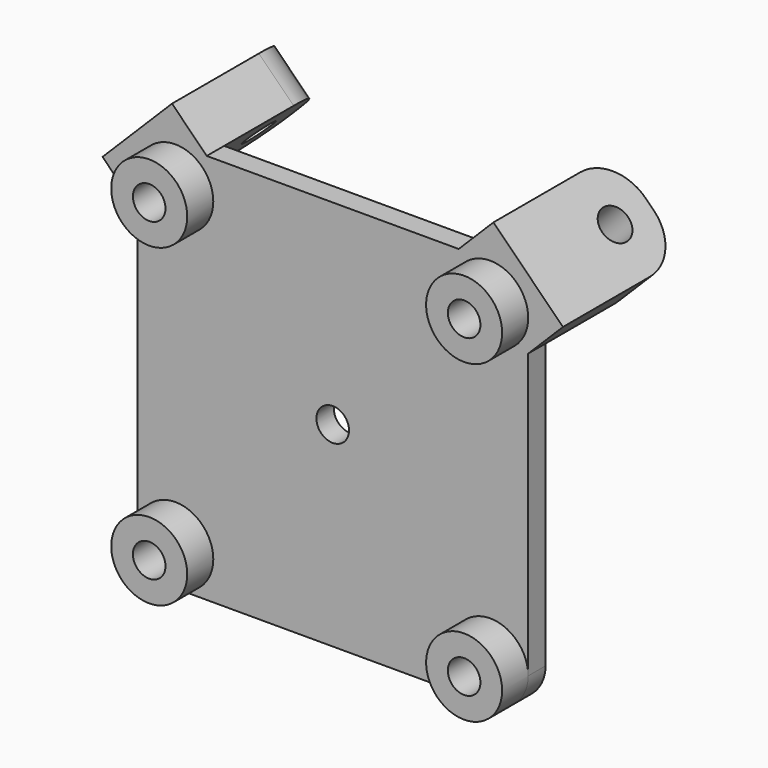
from build123d import *

# Parameters (mm, degrees)
F0_W         = 36
F0_H         = 36
F1_DEPTH     = 2
F2_R         = 3.5
F2_R_2       = 1.5
F3_DEPTH     = 3
F3_FACE_R    = 1.5
F4_R         = 1.5
F5_DEPTH     = 2
F7_DEPTH     = 12
F9_DEPTH     = 2
F10_R        = 1.5
F11_DEPTH    = 4.5254833996
F12_R        = 1.5
F13_DEPTH    = 4.5254833996
F14_R        = 4
F15_T1_DEPTH = 19.4995000071


# Not quite as in the source:
# - a fillet or chamfer that OpenCascade refuses, or shapes differently, is made with other operations: its cross-section is extruded or revolved along the edge and cut away or added


with BuildPart() as f1:
    # F0 (on Front) → F1 (new body)
    with BuildSketch(Plane.XZ):
        with Locations((18, 18)):
            Rectangle(F0_W, F0_H)
    extrude(amount=F1_DEPTH)

    # F2 (on face) → F3 (join)
    with BuildSketch(Plane.XZ.offset(2)):
        with Locations((3.5, 32.5)):
            Circle(F2_R)
        with Locations((3.5, 32.5)):
            Circle(F2_R_2, mode=Mode.SUBTRACT)
        with Locations((32.5, 32.5)):
            Circle(F2_R)
        with Locations((32.5, 32.5)):
            Circle(F2_R_2, mode=Mode.SUBTRACT)
        with Locations((32.5, 3.5)):
            Circle(F2_R)
        with Locations((32.5, 3.5)):
            Circle(F2_R_2, mode=Mode.SUBTRACT)
        with Locations((3.5, 3.5)):
            Circle(F2_R)
        with Locations((3.5, 3.5)):
            Circle(F2_R_2, mode=Mode.SUBTRACT)
    extrude(amount=F3_DEPTH)

    # F3_face (on face) + F4 (on face) → F5 (cut, through all)
    with BuildSketch(Plane(origin=(18, -2, 18), x_dir=(1, 0, 0), z_dir=(0, -1, 0))):
        with Locations((-14.5, 14.5)):
            Circle(F3_FACE_R)
        with Locations((-14.5, -14.5)):
            Circle(F3_FACE_R)
        with Locations((14.5, -14.5)):
            Circle(F3_FACE_R)
        with Locations((14.5, 14.5)):
            Circle(F3_FACE_R)
    with BuildSketch(Plane.XZ.offset(2)):
        with Locations((18, 18)):
            Circle(F4_R)
    extrude(amount=-F5_DEPTH, mode=Mode.SUBTRACT)

    # F6 (on face) → F7 (join)
    with BuildSketch(Plane(origin=(0, 0, 0), x_dir=(-1, 0, 0), z_dir=(0, 1, 0))):
        Polygon((-39.2, 32.8), (-36, 29.6), (-29.6, 36), (-32.8, 39.2), align=None)
        Polygon((-6.4, 36), (0, 29.6), (3.2, 32.8), (-3.2, 39.2), align=None)
    extrude(amount=F7_DEPTH)

    # F9 (add, through all): faces of the model
    f9_faces = [f1.faces().sort_by_distance(p)[0] for p in [
        (37.0666666667, 0, 32.8),
        (32.8, 0, 37.0666666667),
        (3.2, 0, 37.0666666667),
        (-1.0666666667, 0, 32.8),
    ]]
    extrude(f9_faces, amount=F9_DEPTH)

    # F10 (on face) → F11 (cut, through all)
    with BuildSketch(Plane(origin=(32.8, 0, 32.8), x_dir=(0.7071067812, 0, -0.7071067812), z_dir=(-0.7071067812, 0, -0.7071067812))):
        with Locations((0, -8)):
            Circle(F10_R)
    extrude(amount=-F11_DEPTH, mode=Mode.SUBTRACT)

    # F12 (on face) → F13 (cut, through all)
    with BuildSketch(Plane(origin=(-14.8, 0, 14.8), x_dir=(0.7071067812, 0, 0.7071067812), z_dir=(0.7071067812, 0, -0.7071067812))):
        with Locations((25.4558441227, -8)):
            Circle(F12_R)
    extrude(amount=-F13_DEPTH, mode=Mode.SUBTRACT)

    # F14
    f14_edges = [f1.edges().sort_by_distance(p)[0] for p in [
        (-1.6, 12, 31.2),
        (4.8, 12, 37.6),
        (31.2, 12, 37.6),
        (37.6, 12, 31.2),
    ]]
    fillet(f14_edges, radius=F14_R)

    # F15: fillet of radius 3.5 on 2 edges, made by hand

    # F15_s2 → F15_t1 (cut)
    with BuildSketch(Plane.XZ.offset(-8.7497500036)):
        with BuildLine():
            ThreePointArc((-0.0001, 3.4999), (1.0250262658, 1.0250262658), (3.4999, -0.0001))
            Line((3.4999, -0.0001), (3.4999, -0.0701))
            ThreePointArc((3.4999, -0.0701), (1.74995, -0.07), (0, -0.07))
            Line((0, -0.07), (-0.07, 0))
            ThreePointArc((-0.07, 0), (-0.07, 1.74995), (-0.0701, 3.4999))
            Line((-0.0701, 3.4999), (-0.0001, 3.4999))
        make_face()
        with BuildLine():
            ThreePointArc((32.5001, -0.0001), (34.9749737342, 1.0250262658), (36.0001, 3.4999))
            Line((36.0001, 3.4999), (36.0701, 3.4999))
            ThreePointArc((36.0701, 3.4999), (36.07, 1.74995), (36.07, 0))
            Line((36.07, 0), (36, -0.07))
            ThreePointArc((36, -0.07), (34.25005, -0.07), (32.5001, -0.0701))
            Line((32.5001, -0.0701), (32.5001, -0.0001))
        make_face()
    extrude(amount=F15_T1_DEPTH, mode=Mode.SUBTRACT)


solid = f1.part
